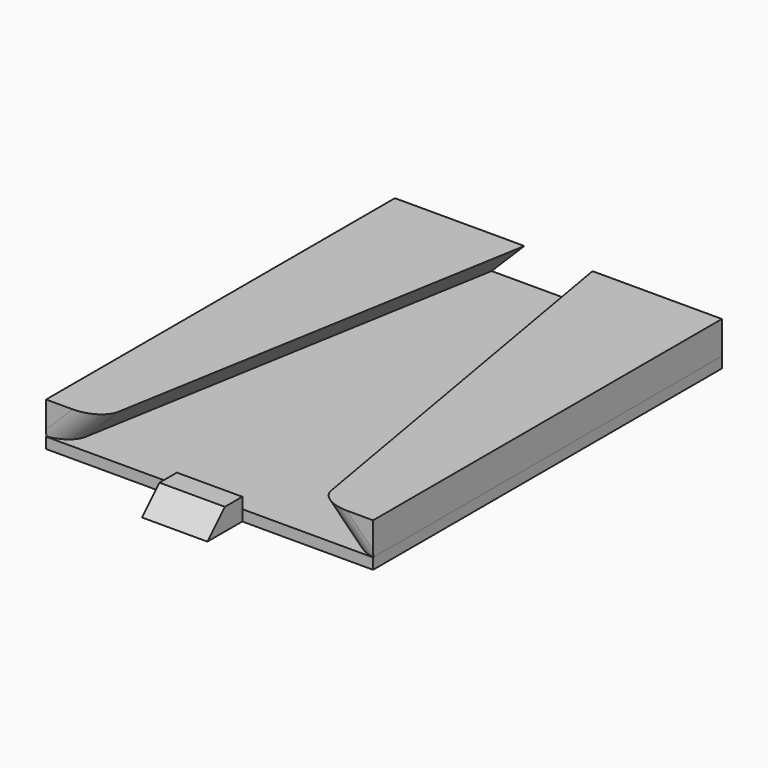
from build123d import *

# Parameters (mm, degrees)
F1_DEPTH     = 200
F2_T1_DEPTH  = 1079.6863395878
F3_R         = 10
F4_W         = 150
F4_H         = 5
F5_DEPTH     = 200
F8_W         = 30
F8_H         = 5
F9_DEPTH     = 25
F10_T1_DEPTH = 107.150489639


# Not quite as in the source:
# - a fillet or chamfer that OpenCascade refuses, or shapes differently, is made with other operations: its cross-section is extruded or revolved along the edge and cut away or added
# - a feature names something its author has since deleted; it is built from what else it names


with BuildPart() as f1:
    # F0 (on Front) → F1 (new body)
    with BuildSketch(Plane.XZ):
        Polygon((-45, 0), (0, 0), (0, 15), (-60, 15), (-52.5, 7.5), align=None)
    extrude(amount=F1_DEPTH)

    # F2: chamfer of 25 x 203.6086606994 on 1 edges, made by hand

    # F2_s2 → F2_t1 (cut)
    with BuildSketch(Plane(origin=(351.7267661385, 0, -351.7267661385), x_dir=(0, 1, 0), z_dir=(-0.7071067812, 0, 0.7071067812))):
        Polygon((-200, 6.8198051534), (3.6086606994, 31.8198051534), (-200, 31.8198051534), align=None)
    extrude(amount=F2_T1_DEPTH, mode=Mode.SUBTRACT)

    # F3
    f3_edges = [f1.edges().sort_by_distance(p)[0] for p in [
        (-17.144661, -200, 7.5),
    ]]
    fillet(f3_edges, radius=F3_R)


with BuildPart() as f5:
    # F4 (on Front) → F5 (new body)
    with BuildSketch(Plane.XZ):
        with Locations((-75, -2.5)):
            Rectangle(F4_W, F4_H)
    extrude(amount=F5_DEPTH)

    # F8 (on face) → F9 (join)
    with BuildSketch(Plane.XZ.offset(200)):
        with Locations((-75, -2.5)):
            Rectangle(F8_W, F8_H)
        with Locations((-75, 2.5)):
            Rectangle(F8_W, F8_H)
    extrude(amount=F9_DEPTH)

    # F10: chamfer of 15 on 1 edges, made by hand

    # F10_s2 → F10_t1 (cut)
    with BuildSketch(Plane.YZ.offset(-128.5752448195)):
        Polygon((-225, -10), (-210, 5), (-225, 5), align=None)
    extrude(amount=F10_T1_DEPTH, mode=Mode.SUBTRACT)


with BuildPart() as f7_1:
    # F7: instance of F1
    add(f1.part.mirror(Plane.YZ.offset(-75)))


solid = Compound([f1.part, f5.part, f7_1.part])
